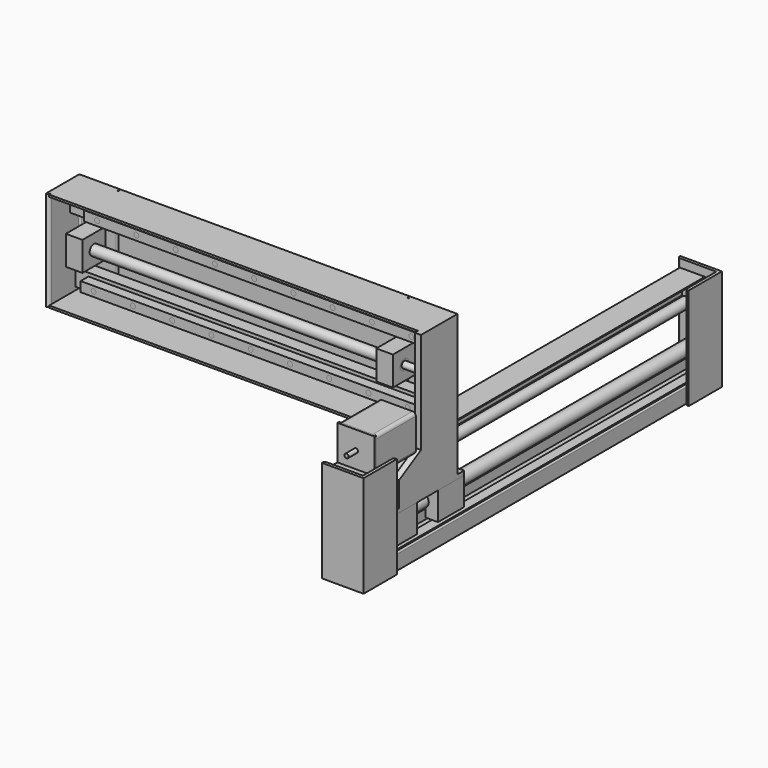
from build123d import *

# Parameters (mm, degrees)
F0_W           = 44.704
F0_H           = 20.352
F1_DEPTH       = 675
F3_DEPTH       = 152.4
F3_DEPTH_BACK  = 3.048
F5_START       = -10
F4_R           = 10
F5_DEPTH       = 630
F7_DEPTH       = 152.4
F7_DEPTH_BACK  = 3.048
F9_DEPTH       = 675
F11_START      = -470
F10_W          = 48
F10_H          = 42.719
F10_R          = 10
F11_DEPTH      = 50
F12_START      = -89.7
F11_FACE_W     = 48
F11_FACE_H     = 42.719
F11_FACE_R     = 10
F12_DEPTH      = 50
F13_START      = -470
F13_DEPTH      = 139.7
F14_W          = 9.525
F14_H          = 112
F15_DEPTH      = 215.9
F16_START      = -10
F10_R_2        = 8
F16_DEPTH      = 650
F17_START      = -497
F17_DEPTH      = 48
F19_DEPTH      = 9.525
F20_W          = 56.4
F20_H          = 25
F21_DEPTH      = 3.175
F22_W          = 56.4
F22_H          = 3.175
F23_DEPTH      = 53.225
F24_R          = 3.175
F25_DEPTH      = 21
F24_R_2        = 2.55
F26_DEPTH      = 76
F28_DEPTH      = 152.4
F29_W          = 4.7625
F29_H          = 152.4
F30_DEPTH      = 441.35
F32_DEPTH      = 152.4
F33_W          = 503.0166667898
F33_H          = 25.4
F33_W_2        = 50.8083332102
F34_DEPTH      = 19.05
F33_W_3        = 494.6916667898
F35_W          = 520
F35_H          = 15
F36_DEPTH      = 15
F37_R          = 3.75
F38_DEPTH      = 15
F39_W          = 25.4
F39_H          = 44.45
F39_W_2        = 14.5916667898
F39_W_3        = 10.8083332102
F40_DEPTH      = 44.45
F41_R          = 8
F41_R_2        = 5
F42_DEPTH      = 480
F43_DEPTH      = 511
F43_DEPTH_BACK = 39
F44_W          = 15
F44_H          = 25.4
F45_DEPTH      = 5
F46_W          = 58.7375
F46_H          = 3.175
F46_W_2        = 59.7749971867
F47_DEPTH      = 560


with BuildPart() as f1:
    # F0 (on Front) → F1 (new body)
    with BuildSketch(Plane.XZ):
        with BuildLine():
            ThreePointArc((198.8949199773, 2), (199.4807064149, 0.5857864376), (200.8949199773, 0))
            Line((200.8949199773, 0), (247.6949199773, 0))
            ThreePointArc((247.6949199773, 0), (249.1091335397, 0.5857864376), (249.6949199773, 2))
            Line((249.6949199773, 2), (249.6949199773, 23.4))
            ThreePointArc((249.6949199773, 23.4), (249.1091335397, 24.8142135624), (247.6949199773, 25.4))
            Line((247.6949199773, 25.4), (200.8949199773, 25.4))
            ThreePointArc((200.8949199773, 25.4), (199.4807064149, 24.8142135624), (198.8949199773, 23.4))
            Line((198.8949199773, 23.4), (198.8949199773, 2))
        make_face()
        with Locations((224.2949199773, 13.224)):
            Rectangle(F0_W, F0_H, mode=Mode.SUBTRACT)
    extrude(amount=F1_DEPTH)


with BuildPart() as f3:
    # F2 (on face) → F3 (new body, two sides)
    with BuildSketch(Plane.XY.offset(3.048)) as f3_sk:
        with BuildLine():
            Line((201.9429199773, -675), (193.9574199773, -675))
            ThreePointArc((193.9574199773, -675), (191.8360996337, -675.8786796564), (190.9574199773, -678))
            Line((190.9574199773, -678), (190.9574199773, -679.7625))
            Line((190.9574199773, -679.7625), (254.4574199773, -679.7625))
            Line((254.4574199773, -679.7625), (254.4574199773, -616.2625))
            Line((254.4574199773, -616.2625), (252.6949199773, -616.2625))
            ThreePointArc((252.6949199773, -616.2625), (250.5735996337, -617.1411796564), (249.6949199773, -619.2625))
            Line((249.6949199773, -619.2625), (249.6949199773, -675))
            Line((249.6949199773, -675), (246.6469199773, -675))
            Line((246.6469199773, -675), (201.9429199773, -675))
        make_face()
    extrude(amount=F3_DEPTH)
    extrude(f3_sk.sketch, amount=-F3_DEPTH_BACK)


with BuildPart() as f5:
    # F4 (on face) → F5 (new body)
    with BuildSketch(Plane(origin=(0, 0, 0), x_dir=(-1, 0, 0), z_dir=(0, 1, 0)).offset(F5_START)):
        with Locations((-224.2949199773, 55.4100826675)):
            Circle(F4_R)
    extrude(amount=-F5_DEPTH)


with BuildPart() as f5b:
    # F4 (on face) → F5, piece 2 (new body)
    with BuildSketch(Plane(origin=(0, 0, 0), x_dir=(-1, 0, 0), z_dir=(0, 1, 0)).offset(F5_START)):
        Polygon((-246.7949199773, 27.4), (-246.7949199773, 25.4), (-201.7949199773, 25.4), (-201.7949199773, 27.4), (-216.7949199773, 27.4), (-219.3114775516, 30.7205021173), (-219.3114775516, 45.4), (-229.3114775516, 45.4), (-229.3114775516, 30.9699550062), (-231.7949199773, 27.4), align=None)
    extrude(amount=-F5_DEPTH)


with BuildPart() as f7:
    # F6 (on face) → F7 (new body, two sides)
    with BuildSketch(Plane.XY.offset(3.048)) as f7_sk:
        with BuildLine():
            ThreePointArc((191.0028244299, 2.9258017551), (191.906983665, 0.8526068438), (194.0019067263, 0))
            Line((194.0019067263, 0), (201.9429199773, 0))
            Line((201.9429199773, 0), (246.6469199773, 0))
            Line((246.6469199773, 0), (249.6949199773, 0))
            Line((249.6949199773, 0), (249.6949199773, -55.7389568545))
            ThreePointArc((249.6949199773, -55.7389568545), (250.5735996337, -57.8602771981), (252.6949199773, -58.7389568545))
            Line((252.6949199773, -58.7389568545), (254.4574199773, -58.7389568545))
            Line((254.4574199773, -58.7389568545), (254.4574199773, 4.7610431455))
            Line((254.4574199773, 4.7610431455), (190.9574199773, 4.7610431455))
            Line((190.9574199773, 4.7610431455), (191.0028244299, 2.9258017551))
        make_face()
    extrude(amount=F7_DEPTH)
    extrude(f7_sk.sketch, amount=-F7_DEPTH_BACK)

    # F8 (on face) → F9 (join)
    with BuildSketch(Plane.XZ):
        with BuildLine():
            Line((232.1019067263, 142.875), (194.1349199773, 142.875))
            Line((194.1349199773, 142.875), (194.1349199773, 104.775))
            Line((194.1349199773, 104.775), (194.2371480266, 104.7725505623))
            ThreePointArc((194.2371480266, 104.7725505623), (196.404768641, 105.6251130976), (197.3090089751, 107.7716897728))
            Line((197.3090089751, 107.7716897728), (197.3090089751, 136.7))
            ThreePointArc((197.3090089751, 136.7), (198.1876886315, 138.8213203436), (200.3090089751, 139.7))
            Line((200.3090089751, 139.7), (229.1019067263, 139.7))
            ThreePointArc((229.1019067263, 139.7), (231.2232270699, 140.5786796564), (232.1019067263, 142.7))
            Line((232.1019067263, 142.7), (232.1019067263, 142.875))
        make_face()
    extrude(amount=F9_DEPTH)


with BuildPart() as f11:
    # F10 (on face) → F11 (new body)
    with BuildSketch(Plane(origin=(0, -10, 0), x_dir=(-1, 0, 0), z_dir=(0, 1, 0)).offset(F11_START)):
        with Locations((-224.2949199773, 54.8371332088)):
            Rectangle(F10_W, F10_H)
        with Locations((-224.2949199773, 55.4100826675)):
            Circle(F10_R, mode=Mode.SUBTRACT)
    extrude(amount=-F11_DEPTH)


with BuildPart() as f12:
    # F11_face (on face) → F12 (new body)
    with BuildSketch(Plane(origin=(224.2949199773, -480, 54.7334691448), x_dir=(-1, 0, 0), z_dir=(0, 1, 0)).offset(F12_START)):
        with Locations((0, 0.103664064)):
            Rectangle(F11_FACE_W, F11_FACE_H)
        with Locations((0, 0.6766135226)):
            Circle(F11_FACE_R, mode=Mode.SUBTRACT)
    extrude(amount=-F12_DEPTH)


with BuildPart() as f13:
    # F10 (on face) → F13 (new body)
    with BuildSketch(Plane(origin=(0, -10, 0), x_dir=(-1, 0, 0), z_dir=(0, 1, 0)).offset(F13_START)):
        Polygon((-248.2949199773, 82.5466332088), (-248.2949199773, 76.1966332088), (-200.2949199773, 76.1966332088), (-197.4949199773, 76.1966332088), (-197.4949199773, 82.5466332088), align=None)
    extrude(amount=-F13_DEPTH)

    # F14 (on face) → F15 (join)
    with BuildSketch(Plane.XY.offset(82.5466332088)):
        with Locations((243.5324199773, -548.7)):
            Rectangle(F14_W, F14_H)
    extrude(amount=F15_DEPTH)

    # F18 (on face) → F19 (cut)
    with BuildSketch(Plane.YZ.offset(248.2949199773)):
        Polygon((-604.7, 298.4466332088), (-604.7, 119.9353337288), (-562.3939633369, 143.7013298273), (-562.3939633369, 298.4466332088), align=None)
    extrude(amount=-F19_DEPTH, mode=Mode.SUBTRACT)

    # F27 (on face) → F28 (join)
    with BuildSketch(Plane.XY.offset(298.4466332088)):
        with BuildLine():
            Line((238.7699199773, -556.2), (238.7699199773, -492.7))
            Line((238.7699199773, -492.7), (175.2699199773, -492.7))
            Line((175.2699199773, -492.7), (175.2699199773, -494.5333332102))
            ThreePointArc((175.2699199773, -494.5333332102), (176.1278530668, -496.6045669105), (178.1990867671, -497.4625))
            Line((178.1990867671, -497.4625), (229.0074199773, -497.4625))
            ThreePointArc((229.0074199773, -497.4625), (232.5429538832, -498.9269660941), (234.0074199773, -502.4625))
            Line((234.0074199773, -502.4625), (234.0074199773, -553.4481295041))
            ThreePointArc((234.0074199773, -553.4481295041), (234.8134241846, -555.3939957927), (236.7592904732, -556.2))
            Line((236.7592904732, -556.2), (238.7699199773, -556.2))
        make_face()
    extrude(amount=-F28_DEPTH)

    # F29 (on face) → F30 (join)
    with BuildSketch(Plane(origin=(175.2699199773, 0, 0), x_dir=(0, -1, 0), z_dir=(-1, 0, 0))):
        with Locations((495.08125, 222.2466332088)):
            Rectangle(F29_W, F29_H)
    extrude(amount=F30_DEPTH)

    # F31 (on face) → F32 (join)
    with BuildSketch(Plane.XY.offset(298.4466332088)):
        with BuildLine():
            Line((-266.0800800227, -493.4700633377), (-266.0800800227, -492.7))
            Line((-266.0800800227, -492.7), (-329.5800800227, -492.7))
            Line((-329.5800800227, -492.7), (-329.5800800227, -556.2))
            Line((-329.5800800227, -556.2), (-329.1589422784, -556.2))
            ThreePointArc((-329.1589422784, -556.2), (-326.0891355878, -554.9284444349), (-324.8175800227, -551.8586377443))
            Line((-324.8175800227, -551.8586377443), (-324.8175800227, -500.2143704959))
            ThreePointArc((-324.8175800227, -500.2143704959), (-324.0115758154, -498.2685042073), (-322.0657095268, -497.4625))
            Line((-322.0657095268, -497.4625), (-270.072516685, -497.4625))
            ThreePointArc((-270.072516685, -497.4625), (-267.2494376476, -496.2931423751), (-266.0800800227, -493.4700633377))
        make_face()
    extrude(amount=-F32_DEPTH)

    # F39 (on face) → F40 (join)
    with BuildSketch(Plane.XZ.offset(497.4625)):
        with Locations((-298.0925800227, 222.2466332088)):
            Rectangle(F39_W, F39_H)
        with Locations((170.9032533722, 222.2466332088)):
            Rectangle(F39_W_2, F39_H)
        with Locations((183.6032533722, 222.2466332088)):
            Rectangle(F39_W_3, F39_H)
    extrude(amount=F40_DEPTH)

    # F44 (on face) → F45 (cut)
    with BuildSketch(Plane.XZ.offset(497.4625)):
        with Locations((215.5074199773, 222.25)):
            Rectangle(F44_W, F44_H)
    extrude(amount=-F45_DEPTH, mode=Mode.SUBTRACT)

    # F46 (on face) → F47 (join)
    with BuildSketch(Plane.YZ.offset(-324.8175800227)):
        with Locations((-526.83125, 296.8591332088)):
            Rectangle(F46_W, F46_H)
        with Locations((-526.3125014067, 147.6341332088)):
            Rectangle(F46_W_2, F46_H)
    extrude(amount=F47_DEPTH)


with BuildPart() as f16:
    # F10 (on face) → F16 (new body)
    with BuildSketch(Plane(origin=(0, -10, 0), x_dir=(-1, 0, 0), z_dir=(0, 1, 0)).offset(F16_START)):
        with Locations((-218.7699199773, 112.5466332088)):
            Circle(F10_R_2)
    extrude(amount=-F16_DEPTH)


with BuildPart() as f17:
    # F10 (on face) → F17 (new body)
    with BuildSketch(Plane(origin=(0, -10, 0), x_dir=(-1, 0, 0), z_dir=(0, 1, 0)).offset(F17_START)):
        with BuildLine():
            ThreePointArc((-198.7699199773, 124.5466332088), (-202.2846386031, 133.0319145831), (-210.7699199773, 136.5466332088))
            Line((-210.7699199773, 136.5466332088), (-226.7699199773, 136.5466332088))
            ThreePointArc((-226.7699199773, 136.5466332088), (-235.2552013515, 133.0319145831), (-238.7699199773, 124.5466332088))
            Line((-238.7699199773, 124.5466332088), (-238.7699199773, 100.5466332088))
            ThreePointArc((-238.7699199773, 100.5466332088), (-235.2552013515, 92.0613518346), (-226.7699199773, 88.5466332088))
            Line((-226.7699199773, 88.5466332088), (-210.7699199773, 88.5466332088))
            ThreePointArc((-210.7699199773, 88.5466332088), (-202.2846386031, 92.0613518346), (-198.7699199773, 100.5466332088))
            Line((-198.7699199773, 100.5466332088), (-198.7699199773, 124.5466332088))
        make_face()
        with Locations((-218.7699199773, 112.5466332088)):
            Circle(F10_R_2, mode=Mode.SUBTRACT)
    extrude(amount=-F17_DEPTH)


with BuildPart() as f21:
    # F20 (on face) → F21 (new body)
    with BuildSketch(Plane.XY.offset(142.875)):
        with Locations((221.4949199773, -662.5)):
            Rectangle(F20_W, F20_H)
    extrude(amount=F21_DEPTH)


with BuildPart() as f23:
    # F22 (on face) → F23 (new body)
    with BuildSketch(Plane.XY.offset(146.05)):
        with Locations((221.4949199773, -651.5875)):
            Rectangle(F22_W, F22_H)
    extrude(amount=F23_DEPTH)

    # F24 (on face) → F25 (join)
    with BuildSketch(Plane(origin=(0, -650, 0), x_dir=(-1, 0, 0), z_dir=(0, 1, 0))):
        with Locations((-221.4949199773, 171.075)):
            Circle(F24_R)
    extrude(amount=-F25_DEPTH)


with BuildPart() as f26:
    # F24 (on face) → F26 (new body)
    with BuildSketch(Plane(origin=(0, -650, 0), x_dir=(-1, 0, 0), z_dir=(0, 1, 0))):
        with BuildLine():
            Line((-198.2949199773, 199.275), (-244.6949199773, 199.275))
            ThreePointArc((-244.6949199773, 199.275), (-248.2304538832, 197.8105339059), (-249.6949199773, 194.275))
            Line((-249.6949199773, 194.275), (-249.6949199773, 147.875))
            ThreePointArc((-249.6949199773, 147.875), (-248.2304538832, 144.3394660941), (-244.6949199773, 142.875))
            Line((-244.6949199773, 142.875), (-198.2949199773, 142.875))
            ThreePointArc((-198.2949199773, 142.875), (-194.7593860714, 144.3394660941), (-193.2949199773, 147.875))
            Line((-193.2949199773, 147.875), (-193.2949199773, 194.275))
            ThreePointArc((-193.2949199773, 194.275), (-194.7593860714, 197.8105339059), (-198.2949199773, 199.275))
        make_face()
        with Locations((-243.1900054216, 147.505)):
            Circle(F24_R_2, mode=Mode.SUBTRACT)
        with Locations((-221.4949199773, 171.075)):
            Circle(F24_R, mode=Mode.SUBTRACT)
        with Locations((-197.9249199773, 147.505)):
            Circle(F24_R_2, mode=Mode.SUBTRACT)
        with Locations((-245.0649199773, 194.645)):
            Circle(F24_R_2, mode=Mode.SUBTRACT)
        with Locations((-197.9249199773, 194.645)):
            Circle(F24_R_2, mode=Mode.SUBTRACT)
    extrude(amount=F26_DEPTH)


with BuildPart() as f34:
    # F33 (on face) → F34 (new body)
    with BuildSketch(Plane.XZ.offset(497.4625)):
        with Locations((-73.3092466278, 270.7466332088)):
            Rectangle(F33_W, F33_H)
        with Locations((203.6032533722, 270.7466332088)):
            Rectangle(F33_W_2, F33_H)
    extrude(amount=F34_DEPTH)


with BuildPart() as f34b:
    # F33 (on face) → F34, piece 2 (new body)
    with BuildSketch(Plane.XZ.offset(497.4625)):
        with Locations((203.6032533722, 173.7466332088)):
            Rectangle(F33_W_2, F33_H)
        with Locations((-69.1467466278, 173.7466332088)):
            Rectangle(F33_W_3, F33_H)
    extrude(amount=F34_DEPTH)


with BuildPart() as f36:
    # F35 (on face) → F36 (new body)
    with BuildSketch(Plane.XZ.offset(516.5125)):
        with Locations((-31.3917899132, 270.7466332088)):
            Rectangle(F35_W, F35_H)
    extrude(amount=F36_DEPTH)


with BuildPart() as f36b:
    # F35 (on face) → F36, piece 2 (new body)
    with BuildSketch(Plane.XZ.offset(516.5125)):
        with Locations((-36.6336607933, 173.7466332088)):
            Rectangle(F35_W, F35_H)
    extrude(amount=F36_DEPTH)


with BuildPart() as f38:
    # F37 (on face) → F38 (new body)
    with BuildSketch(Plane.XZ.offset(531.5125)):
        with Locations((-271.3917899132, 270.7466332088)):
            Circle(F37_R)
    extrude(amount=-F38_DEPTH)


with BuildPart() as f38b:
    # F37 (on face) → F38, piece 2 (new body)
    with BuildSketch(Plane.XZ.offset(531.5125)):
        with Locations((-211.3917899132, 270.7466332088)):
            Circle(F37_R)
    extrude(amount=-F38_DEPTH)


with BuildPart() as f38c:
    # F37 (on face) → F38, piece 3 (new body)
    with BuildSketch(Plane.XZ.offset(531.5125)):
        with Locations((-151.3917899132, 270.7466332088)):
            Circle(F37_R)
    extrude(amount=-F38_DEPTH)


with BuildPart() as f38d:
    # F37 (on face) → F38, piece 4 (new body)
    with BuildSketch(Plane.XZ.offset(531.5125)):
        with Locations((-91.3917899132, 270.7466332088)):
            Circle(F37_R)
    extrude(amount=-F38_DEPTH)


with BuildPart() as f38e:
    # F37 (on face) → F38, piece 5 (new body)
    with BuildSketch(Plane.XZ.offset(531.5125)):
        with Locations((-31.3917899132, 270.7466332088)):
            Circle(F37_R)
    extrude(amount=-F38_DEPTH)


with BuildPart() as f38f:
    # F37 (on face) → F38, piece 6 (new body)
    with BuildSketch(Plane.XZ.offset(531.5125)):
        with Locations((28.6082100868, 270.7466332088)):
            Circle(F37_R)
    extrude(amount=-F38_DEPTH)


with BuildPart() as f38g:
    # F37 (on face) → F38, piece 7 (new body)
    with BuildSketch(Plane.XZ.offset(531.5125)):
        with Locations((88.6082100868, 270.7466332088)):
            Circle(F37_R)
    extrude(amount=-F38_DEPTH)


with BuildPart() as f38h:
    # F37 (on face) → F38, piece 8 (new body)
    with BuildSketch(Plane.XZ.offset(531.5125)):
        with Locations((148.6082100868, 270.7466332088)):
            Circle(F37_R)
    extrude(amount=-F38_DEPTH)


with BuildPart() as f38i:
    # F37 (on face) → F38, piece 9 (new body)
    with BuildSketch(Plane.XZ.offset(531.5125)):
        with Locations((208.6082100868, 270.7466332088)):
            Circle(F37_R)
    extrude(amount=-F38_DEPTH)


with BuildPart() as f38j:
    # F37 (on face) → F38, piece 10 (new body)
    with BuildSketch(Plane.XZ.offset(531.5125)):
        with Locations((203.3663392067, 173.7466332088)):
            Circle(F37_R)
    extrude(amount=-F38_DEPTH)


with BuildPart() as f38k:
    # F37 (on face) → F38, piece 11 (new body)
    with BuildSketch(Plane.XZ.offset(531.5125)):
        with Locations((143.3663392067, 173.7466332088)):
            Circle(F37_R)
    extrude(amount=-F38_DEPTH)


with BuildPart() as f38l:
    # F37 (on face) → F38, piece 12 (new body)
    with BuildSketch(Plane.XZ.offset(531.5125)):
        with Locations((83.3663392067, 173.7466332088)):
            Circle(F37_R)
    extrude(amount=-F38_DEPTH)


with BuildPart() as f38m:
    # F37 (on face) → F38, piece 13 (new body)
    with BuildSketch(Plane.XZ.offset(531.5125)):
        with Locations((23.3663392067, 173.7466332088)):
            Circle(F37_R)
    extrude(amount=-F38_DEPTH)


with BuildPart() as f38n:
    # F37 (on face) → F38, piece 14 (new body)
    with BuildSketch(Plane.XZ.offset(531.5125)):
        with Locations((-36.6336607933, 173.7466332088)):
            Circle(F37_R)
    extrude(amount=-F38_DEPTH)


with BuildPart() as f38o:
    # F37 (on face) → F38, piece 15 (new body)
    with BuildSketch(Plane.XZ.offset(531.5125)):
        with Locations((-96.6336607933, 173.7466332088)):
            Circle(F37_R)
    extrude(amount=-F38_DEPTH)


with BuildPart() as f38p:
    # F37 (on face) → F38, piece 16 (new body)
    with BuildSketch(Plane.XZ.offset(531.5125)):
        with Locations((-276.6336607933, 173.7466332088)):
            Circle(F37_R)
    extrude(amount=-F38_DEPTH)


with BuildPart() as f38q:
    # F37 (on face) → F38, piece 17 (new body)
    with BuildSketch(Plane.XZ.offset(531.5125)):
        with Locations((-216.6336607933, 173.7466332088)):
            Circle(F37_R)
    extrude(amount=-F38_DEPTH)


with BuildPart() as f38r:
    # F37 (on face) → F38, piece 18 (new body)
    with BuildSketch(Plane.XZ.offset(531.5125)):
        with Locations((-156.6336607933, 173.7466332088)):
            Circle(F37_R)
    extrude(amount=-F38_DEPTH)


with BuildPart() as f42:
    # F41 (on face) → F42 (new body)
    with BuildSketch(Plane.YZ.offset(189.0074199773)):
        with Locations((-520.1998949051, 222.2466332088)):
            Circle(F41_R)
        with Locations((-520.1998949051, 222.2466332088)):
            Circle(F41_R_2, mode=Mode.SUBTRACT)
        with Locations((-520.1998949051, 222.2466332088)):
            Circle(F41_R_2)
    extrude(amount=-F42_DEPTH)


with BuildPart() as f43:
    # F41 (on face) → F43 (new body, two sides)
    with BuildSketch(Plane.YZ.offset(189.0074199773)) as f43_sk:
        with Locations((-520.1998949051, 222.2466332088)):
            Circle(F41_R_2)
    extrude(amount=-F43_DEPTH)
    extrude(f43_sk.sketch, amount=F43_DEPTH_BACK)


solid = Compound([f1.part, f3.part, f5.part, f5b.part, f7.part, f11.part, f12.part, f13.part, f16.part, f17.part, f21.part, f23.part, f26.part, f34.part, f34b.part, f36.part, f36b.part, f38.part, f38b.part, f38c.part, f38d.part, f38e.part, f38f.part, f38g.part, f38h.part, f38i.part, f38j.part, f38k.part, f38l.part, f38m.part, f38n.part, f38o.part, f38p.part, f38q.part, f38r.part, f42.part, f43.part])
